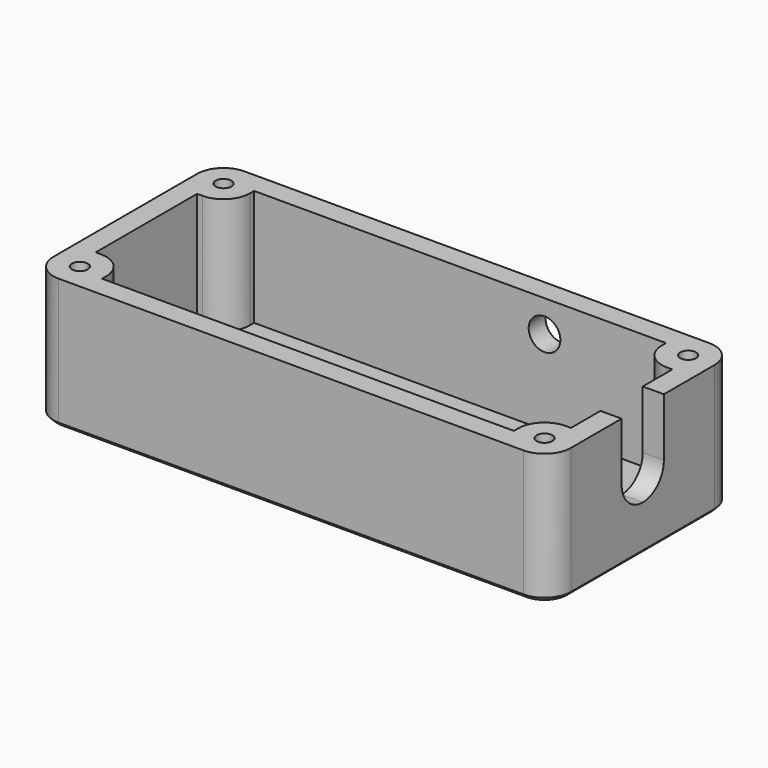
from build123d import *

# Parameters (mm, degrees)
F0_W      = 49
F0_H      = 22
F0_W_2    = 45
F0_H_2    = 18
F1_DEPTH  = 11
F2_W      = 49
F2_H      = 22
F3_DEPTH  = 1.4
F4_W      = 5
F4_H      = 8
F5_DEPTH  = 2
F6_R      = 1.5
F7_DEPTH  = 2
F8_W      = 3
F8_H      = 3
F9_DEPTH  = 11
F10_R     = 2.5
F11_R     = 2.5
F12_R     = 2.49999
F14_D     = 1.5
F14_DEPTH = 8
F14_TIP   = 0.4506454643
F15_SIZE  = 0.4


# Not quite as in the source:
# - a fillet or chamfer is up to 0.001 mm smaller than in the source, because OpenCascade refuses the exact size


with BuildPart() as f1:
    # F0 (on Top) → F1 (new body)
    with BuildSketch(Plane.XY):
        with Locations((22.5, 9)):
            Rectangle(F0_W, F0_H)
        with Locations((22.5, 9)):
            Rectangle(F0_W_2, F0_H_2, mode=Mode.SUBTRACT)
    extrude(amount=F1_DEPTH)

    # F2 (on face) → F3 (join)
    with BuildSketch(Plane(origin=(0, 0, 0), x_dir=(1, 0, 0), z_dir=(0, 0, -1))):
        with Locations((22.5, -9)):
            Rectangle(F2_W, F2_H)
    extrude(amount=F3_DEPTH)

    # F4 (on face) → F5 (cut, through all)
    with BuildSketch(Plane.YZ.offset(47)):
        with Locations((9, 7)):
            Rectangle(F4_W, F4_H)
    extrude(amount=-F5_DEPTH, mode=Mode.SUBTRACT)

    # F6 (on face) → F7 (cut, through all)
    with BuildSketch(Plane(origin=(0, 20, 0), x_dir=(-1, 0, 0), z_dir=(0, 1, 0))):
        with Locations((-30.5, 8)):
            Circle(F6_R)
    extrude(amount=-F7_DEPTH, mode=Mode.SUBTRACT)

    # F8 (on face) → F9 (join, through all)
    with BuildSketch(Plane.XY):
        with Locations((1.5, 1.5)):
            Rectangle(F8_W, F8_H)
        with Locations((43.5, 1.5)):
            Rectangle(F8_W, F8_H)
        with Locations((1.5, 16.5)):
            Rectangle(F8_W, F8_H)
        with Locations((43.5, 16.5)):
            Rectangle(F8_W, F8_H)
    extrude(amount=F9_DEPTH)

    # F10
    f10_edges = [f1.edges().sort_by_distance(p)[0] for p in [
        (42, 3, 5.5),
        (42, 15, 5.5),
        (3, 3, 5.5),
        (3, 15, 5.5),
    ]]
    fillet(f10_edges, radius=F10_R)

    # F11
    f11_edges = [f1.edges().sort_by_distance(p)[0] for p in [
        (47, -2, 4.8),
        (47, 20, 4.8),
        (-2, 20, 4.8),
        (-2, -2, 4.8),
    ]]
    fillet(f11_edges, radius=F11_R)

    # F12 (radius 2.5 in the source; OpenCascade refuses exactly that, so slightly less here)
    f12_edges = [f1.edges().sort_by_distance(p)[0] for p in [
        (46, 11.5, 3),
        (46, 6.5, 3),
    ]]
    fillet(f12_edges, radius=F12_R)

    # F14
    with Locations(Plane.XY.offset(11)):
        with Locations((44.5, 17.5), (44.5, 0.5), (0.5, 0.5), (0.5, 17.5)):
            Hole(F14_D / 2, depth=F14_DEPTH)
            with Locations((0, 0, -(F14_DEPTH + F14_TIP / 2))):  # 118° drill point
                Cone(0, F14_D / 2, F14_TIP, mode=Mode.SUBTRACT)

    # F15
    f15_edges = [f1.edges().sort_by_distance(p)[0] for p in [
        (-2, 9, -1.4),
        (-1.267767, -1.267767, -1.4),
        (-1.267767, 19.267767, -1.4),
        (22.5, -2, -1.4),
        (22.5, 20, -1.4),
        (46.267767, -1.267767, -1.4),
        (46.267767, 19.267767, -1.4),
        (47, 9, -1.4),
    ]]
    chamfer(f15_edges, length=F15_SIZE)


solid = f1.part
